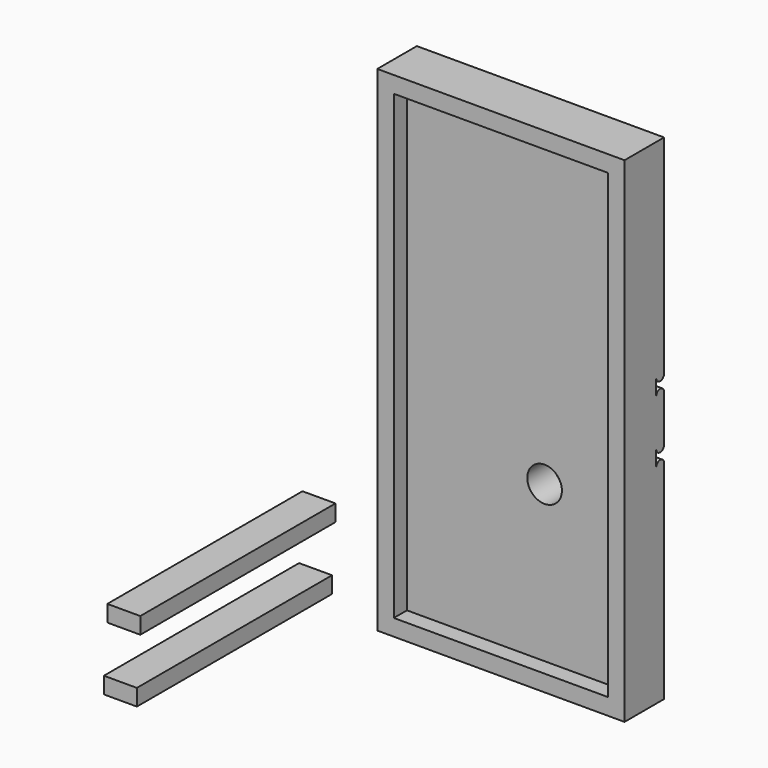
from build123d import *

# Parameters (mm, degrees)
F0_W          = 75
F0_H          = 150
F0_W_2        = 65
F0_H_2        = 140
F1_DEPTH      = 15
F0_R          = 5.25
F2_DEPTH      = 10
F3_W          = 74
F3_H          = 5
F4_DEPTH      = 10
F5_DEPTH      = 37.501
F5_DEPTH_BACK = 37.501


with BuildPart() as f1:
    # F0 (on Front) → F1 (new body)
    with BuildSketch(Plane.XZ):
        Rectangle(F0_W, F0_H)
        Rectangle(F0_W_2, F0_H_2, mode=Mode.SUBTRACT)
    extrude(amount=F1_DEPTH)

    # F0 (on Front) → F2 (join)
    with BuildSketch(Plane.XZ):
        Rectangle(F0_W_2, F0_H_2)
        with Locations((9.25, -22.75)):
            Circle(F0_R, mode=Mode.SUBTRACT)
    extrude(amount=F2_DEPTH)

    # F3 (on Right) → F5 (cut, two sides)
    with BuildSketch(Plane.YZ) as f5_sk:
        with Locations((-127.245810883, 2.5)):
            Rectangle(F3_W, F3_H)
        with Locations((-128.5421704054, -16.1596382409)):
            Rectangle(F3_W, F3_H)
        with BuildLine():
            Line((0, -12), (0, -7))
            ThreePointArc((0, -7), (-1.5, -8.5), (-3, -7))
            Line((-3, -7), (-3, -12))
            ThreePointArc((-3, -12), (-1.5, -10.5), (0, -12))
        make_face()
        with BuildLine():
            ThreePointArc((0, 12), (-1.5, 10.5), (-3, 12))
            Line((-3, 12), (-3, 7))
            ThreePointArc((-3, 7), (-1.5, 8.5), (0, 7))
            Line((0, 7), (0, 12))
        make_face()
    extrude(amount=F5_DEPTH, mode=Mode.SUBTRACT)
    extrude(f5_sk.sketch, amount=-F5_DEPTH_BACK, mode=Mode.SUBTRACT)


with BuildPart() as f4:
    # F3 (on Right) → F4 (new body)
    with BuildSketch(Plane.YZ):
        with Locations((-127.245810883, 2.5)):
            Rectangle(F3_W, F3_H)
    extrude(amount=F4_DEPTH)


with BuildPart() as f4b:
    # F3 (on Right) → F4, piece 2 (new body)
    with BuildSketch(Plane.YZ):
        with Locations((-128.5421704054, -16.1596382409)):
            Rectangle(F3_W, F3_H)
    extrude(amount=F4_DEPTH)


solid = Compound([f1.part, f4.part, f4b.part])
